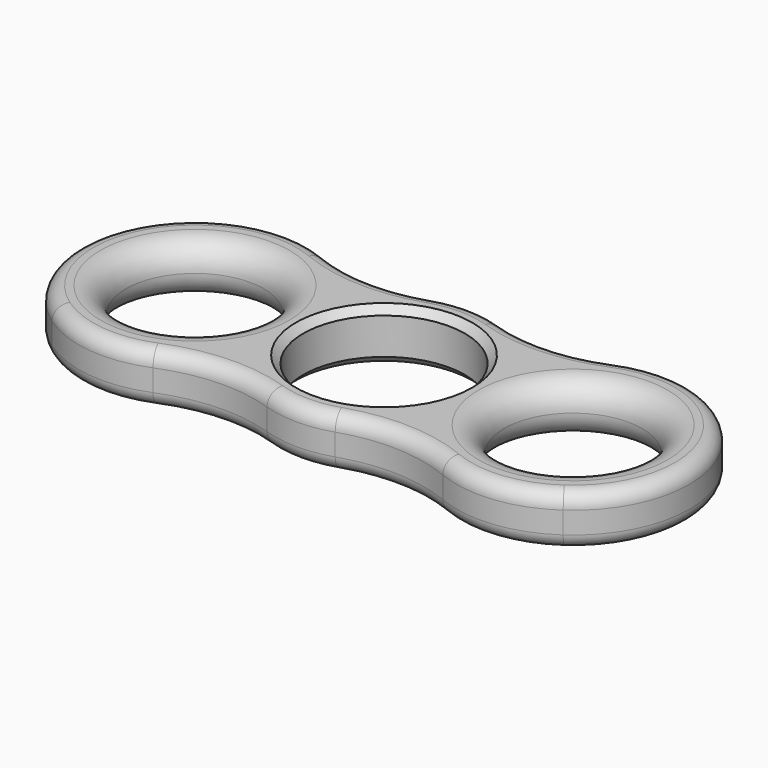
from build123d import *

# Parameters (mm, degrees)
F1_DEPTH = 7
F2_R     = 11.125
F3_DEPTH = 7.001
F4_R     = 2
F5_R     = 9.5
F6_DEPTH = 7.001
F7_R     = 3.49999
F8_SIZE  = 1


# Not quite as in the source:
# - a fillet or chamfer is up to 0.001 mm smaller than in the source, because OpenCascade refuses the exact size


with BuildPart() as f1:
    # F0 (on Top) → F1 (new body)
    with BuildSketch(Plane.XY):
        with BuildLine():
            ThreePointArc((-19.9190283401, -14.7993845707), (-12.3514453516, -13.1628621978), (-4.6855509356, -14.2494074414))
            ThreePointArc((-4.6855509356, -14.2494074414), (0, -15), (4.6855509356, -14.2494074414))
            ThreePointArc((4.6855509356, -14.2494074414), (12.3514453516, -13.1628621978), (19.9190283401, -14.7993845707))
            ThreePointArc((19.9190283401, -14.7993845707), (27.7435994179, -15.9047119141), (35.1428571429, -13.1304289064))
            ThreePointArc((35.1428571429, -13.1304289064), (40.048573091, 7.6575187957), (19.9190283401, 14.7993845707))
            ThreePointArc((19.9190283401, 14.7993845707), (12.3514453516, 13.1628621978), (4.6855509356, 14.2494074414))
            ThreePointArc((4.6855509356, 14.2494074414), (0, 15), (-4.6855509356, 14.2494074414))
            ThreePointArc((-4.6855509356, 14.2494074414), (-12.3514453516, 13.1628621978), (-19.9190283401, 14.7993845707))
            ThreePointArc((-19.9190283401, 14.7993845707), (-40.048573091, 7.6575187957), (-35.1428571429, -13.1304289064))
            ThreePointArc((-35.1428571429, -13.1304289064), (-27.7435994179, -15.9047119141), (-19.9190283401, -14.7993845707))
        make_face()
    extrude(amount=F1_DEPTH)

    # F2 (on face) → F3 (cut, through all)
    with BuildSketch(Plane.XY.offset(7)):
        Circle(F2_R)
    extrude(amount=-F3_DEPTH, mode=Mode.SUBTRACT)

    # F4
    f4_edges = [f1.edges().sort_by_distance(p)[0] for p in [
        (-19.919028, -14.799385, 3.5),
        (-42, 0, 0),
        (-19.919028, 14.799385, 3.5),
        (-42, 0, 7),
        (-4.685551, -14.249407, 3.5),
        (-12.351445, -13.162862, 0),
        (-12.351445, -13.162862, 7),
        (4.685551, -14.249407, 3.5),
        (0, -15, 0),
        (0, -15, 7),
        (19.919028, -14.799385, 3.5),
        (12.351445, -13.162862, 0),
        (12.351445, -13.162862, 7),
        (42, 0, 7),
        (19.919028, 14.799385, 3.5),
        (42, 0, 0),
        (4.685551, 14.249407, 3.5),
        (12.351445, 13.162862, 0),
        (12.351445, 13.162862, 7),
        (-4.685551, 14.249407, 3.5),
        (0, 15, 0),
        (0, 15, 7),
        (-12.351445, 13.162862, 0),
        (-12.351445, 13.162862, 7),
    ]]
    fillet(f4_edges, radius=F4_R)

    # F5 (on face) → F6 (cut, through all)
    with BuildSketch(Plane.XY.offset(7)):
        with Locations((-26, 0)):
            Circle(F5_R)
        with Locations((26, 0)):
            Circle(F5_R)
    extrude(amount=-F6_DEPTH, mode=Mode.SUBTRACT)

    # F7 (radius 3.5 in the source; OpenCascade refuses exactly that, so slightly less here)
    f7_edges = [f1.edges().sort_by_distance(p)[0] for p in [
        (-35.5, 0, 7),
        (-16.5, 0, 3.5),
        (-35.5, 0, 0),
        (16.5, 0, 7),
        (35.5, 0, 3.5),
        (16.5, 0, 0),
    ]]
    fillet(f7_edges, radius=F7_R)

    # F8
    f8_edges = [f1.edges().sort_by_distance(p)[0] for p in [
        (-11.125, 0, 7),
        (11.125, 0, 3.5),
        (-11.125, 0, 0),
    ]]
    chamfer(f8_edges, length=F8_SIZE)


solid = f1.part
